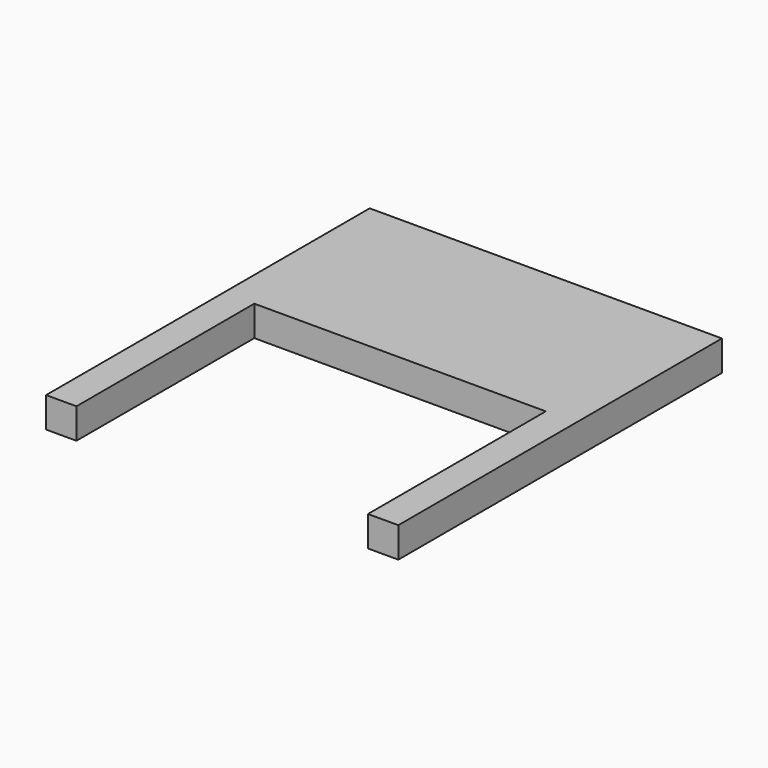
from build123d import *

# Parameters (mm, degrees)
F0_W     = 5
F0_H     = 36.6
F0_W_2   = 5.0038
F1_DEPTH = 5


# Not quite as in the source:
# - the program builds the solid bodies; features that only make, move or delete a surface that nothing else refers to are left out


with BuildPart() as f1:
    # F0 (on Top) → F1 (new body)
    with BuildSketch(Plane.XY):
        Polygon((33.0467298965, 30), (-24.9532701035, 30), (-24.9532701035, 0), (-19.9532701035, 0), (28.0429298965, 0), (33.0467298965, 0), align=None)
        with Locations((-22.4532701035, -18.3)):
            Rectangle(F0_W, F0_H)
        with Locations((30.5448298965, -18.3)):
            Rectangle(F0_W_2, F0_H)
    extrude(amount=F1_DEPTH)


solid = f1.part
